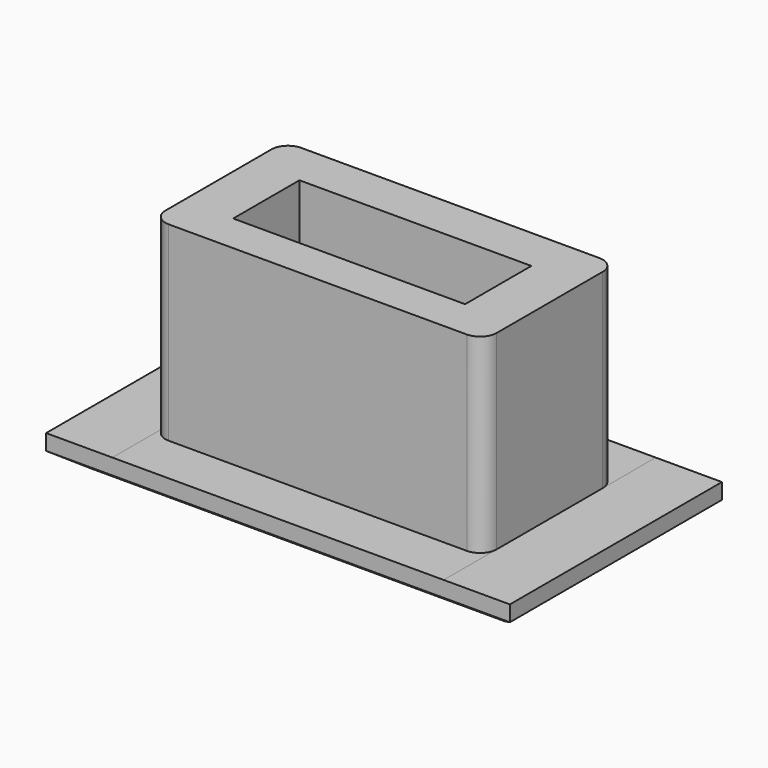
from build123d import *
from build123d import SkipClean  # not in build123d's __all__

# Parameters (mm, degrees)
F0_W     = 20
F0_H     = 11.5
F1_DEPTH = 16
F2_W     = 3
F2_H     = 11.5
F3_DEPTH = 25
F4_W     = 17
F4_H     = 7.5
F4_W_2   = 14
F4_H_2   = 5
F5_DEPTH = 10
F6_DEPTH = 25
F7_SIZE2 = 1.0503113073
F7_SIZE  = 1.5
F8_R     = 1


# Not quite as in the source:
# - ends of sketch curves that miss each other by under 0.0002 mm in the source are joined


with BuildPart() as f1:
    # F0 (on Front) → F1 (new body)
    with BuildSketch(Plane.XZ):
        Rectangle(F0_W, F0_H)
        Polygon((13.9961953573, -5.7499998733), (10, -5.7499998733), (-10, -5.75), (-14.0038046427, -5.7499998733), (-14.0038046427, -7.7499998733), (13.9961953573, -7.7499998733), align=None)
    extrude(amount=-F1_DEPTH)

    # F2 (on face) → F3 (cut)
    with BuildSketch(Plane.YZ.offset(10)):
        with Locations((1.5, 0)):
            Rectangle(F2_W, F2_H)
        with Locations((14.50000076, 0)):
            Rectangle(F2_W, F2_H)
    with SkipClean():  # cleaning this boolean's faces spoils the solid; the shape is the same uncleaned
        extrude(amount=-F3_DEPTH, mode=Mode.SUBTRACT)

    # F4 (on face) → F5 (cut)
    with BuildSketch(Plane(origin=(0, 0, -7.7499998733), x_dir=(1, 0, 0), z_dir=(0, 0, -1))):
        with Locations((0, -7.8641947285)):
            Rectangle(F4_W, F4_H)
        with Locations((0, -7.8641947285)):
            Rectangle(F4_W_2, F4_H_2, mode=Mode.SUBTRACT)
    with SkipClean():  # cleaning this boolean's faces spoils the solid; the shape is the same uncleaned
        extrude(amount=-F5_DEPTH, mode=Mode.SUBTRACT)

    # F4 (on face) → F6 (cut)
    with BuildSketch(Plane(origin=(0, 0, -7.7499998733), x_dir=(1, 0, 0), z_dir=(0, 0, -1))):
        with Locations((0, -7.8641947285)):
            Rectangle(F4_W_2, F4_H_2)
    with SkipClean():  # cleaning this boolean's faces spoils the solid; the shape is the same uncleaned
        extrude(amount=-F6_DEPTH, mode=Mode.SUBTRACT)

    # F7
    f7_edges = [f1.edges().sort_by_distance(p)[0] for p in [
        (-0.003805, 16, -7.75),
        (13.996195, 8, -7.75),
        (-0.003805, 0, -7.75),
        (-14.003805, 8, -7.75),
    ]]
    f7_side = f1.faces().sort_by_distance((-13.681314, 8, -7.75))[0]
    chamfer(f7_edges, length=F7_SIZE, length2=F7_SIZE2, reference=f7_side)

    # F8
    f8_edges = [f1.edges().sort_by_distance(p)[0] for p in [
        (10, 3, 0),
        (10, 13.000001, 0),
        (-10, 3, 0),
        (-10, 13.000001, 0),
    ]]
    fillet(f8_edges, radius=F8_R)


solid = f1.part
